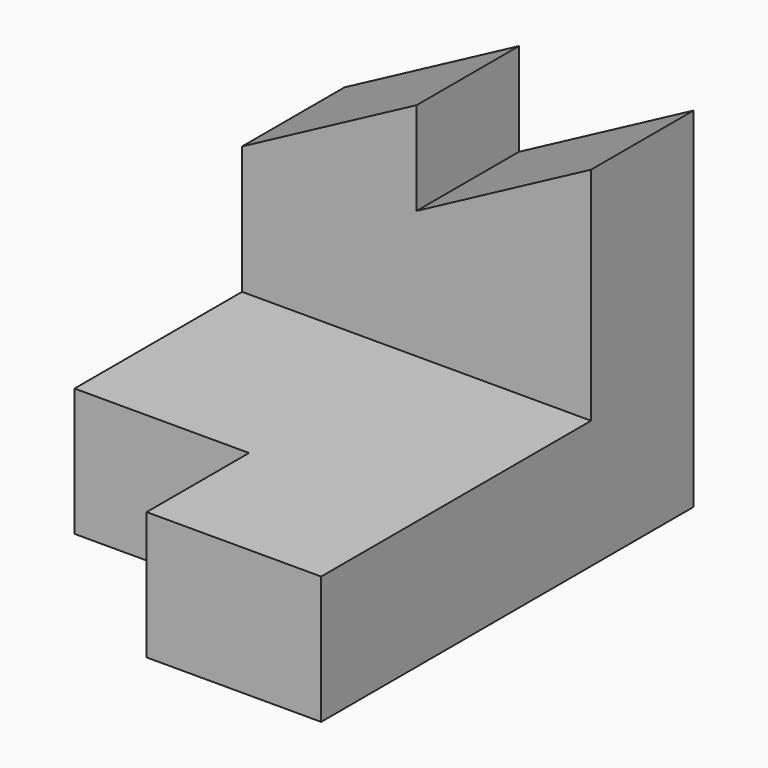
from build123d import *

# Parameters (mm, degrees)
F1_DEPTH  = 30
F2_W      = 11
F2_H      = 15
F3_DEPTH  = 11
F4_W      = 15
F4_H      = 8
F5_DEPTH  = 11
F6_ANGLE  = -90
F8_DEPTH  = 11
F10_DEPTH = 11


with BuildPart() as f1:
    # F0 (on Front) → F1 (new body)
    with BuildSketch(Plane.XZ):
        Polygon((0, 30), (0, 0), (40, 0), (40, 11), (11, 11), (11, 30), align=None)
    extrude(amount=F1_DEPTH)

    # F2 (on face) → F3 (cut, through all)
    with BuildSketch(Plane.XY.offset(11)):
        with Locations((34.5, -22.5)):
            Rectangle(F2_W, F2_H)
    extrude(amount=-F3_DEPTH, mode=Mode.SUBTRACT)

    # F4 (on face) → F5 (cut, through all)
    with BuildSketch(Plane.YZ.offset(11)):
        with Locations((-22.5, 26)):
            Rectangle(F4_W, F4_H)
    extrude(amount=-F5_DEPTH, mode=Mode.SUBTRACT)


with BuildPart() as f1_1:
    # F6: moved
    add(f1.part.rotate(Axis((0, 0, 15), (0, 0, 1)), F6_ANGLE))

    # F7 (on face) → F8 (join, through all)
    with BuildSketch(Plane.XZ.offset(11)):
        Polygon((-15, 22), (-15, 30), (-30, 22), align=None)
    extrude(amount=-F8_DEPTH)

    # F9 (on face) → F10 (cut, through all)
    with BuildSketch(Plane.XZ.offset(11)):
        Polygon((0, 30), (-15, 30), (-15, 22), align=None)
    extrude(amount=-F10_DEPTH, mode=Mode.SUBTRACT)


solid = f1_1.part
